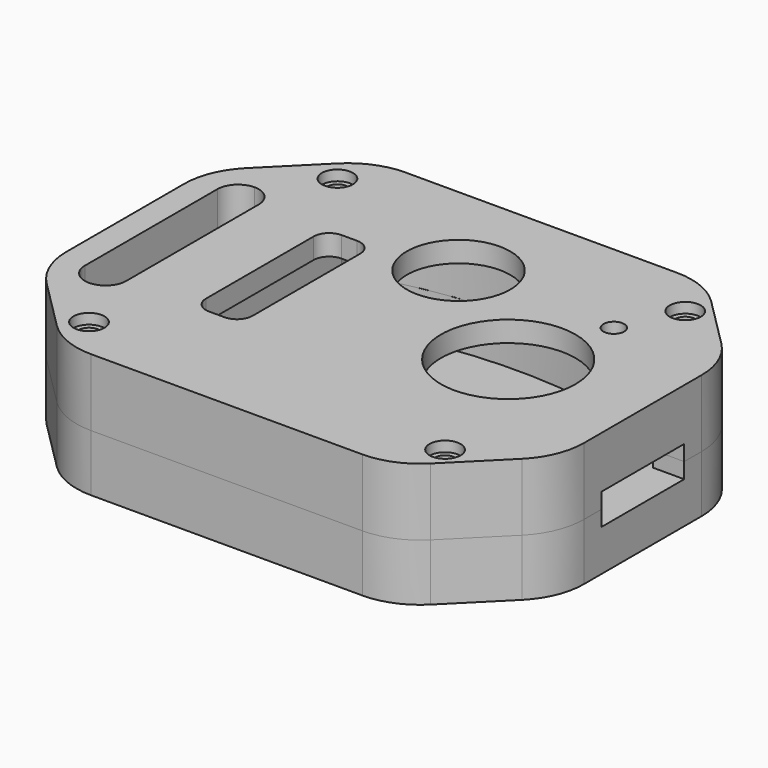
from build123d import *

# Parameters (mm, degrees)
F1_DEPTH   = 5.5
F2_DEPTH   = 1.5
F4_DEPTH   = 4.5
F5_W       = 4
F5_H       = 20
F6_DEPTH   = 25
F7_DEPTH   = 6.5
F8_DEPTH   = 1.5
F9_DEPTH   = 4.5
F10_DEPTH  = 25
F11_R      = 5
F11_R_2    = 6.5
F11_R_3    = 1
F12_DEPTH  = 4
F14_DEPTH  = 4.5
F15_SIZE   = 9
F15_2_SIZE = 9
F16_R      = 7
F16_2_R    = 7
F17_R      = 1.99999
F17_2_R    = 1.99999
F18_R      = 1
F19_DEPTH  = 7.5
F20_R      = 1.5
F20_R_2    = 1
F21_DEPTH  = 1
F22_R      = 1.5
F23_DEPTH  = 1


# Not quite as in the source:
# - a fillet or chamfer is up to 0.001 mm smaller than in the source, because OpenCascade refuses the exact size


with BuildPart() as f1:
    # F0 (on Top) → F1 (new body)
    with BuildSketch(Plane.XY):
        Polygon((25, 5), (25, 19), (-25, 19), (-25, -19), (25, -19), (25, -5), (22, -5), (22, -10), (20.5, -10), (19, -7), (19, 7), (20.5, 10), (22, 10), (22, 5), align=None)
        Polygon((25, -5), (25, 5), (22, 5), (22, 10), (20.5, 10), (19, 7), (19, -7), (20.5, -10), (22, -10), (22, -5), align=None)
    extrude(amount=-F1_DEPTH)

    # F0 (on Top) → F2 (cut)
    with BuildSketch(Plane.XY):
        Polygon((25, -5), (25, 5), (22, 5), (22, 10), (20.5, 10), (19, 7), (19, -7), (20.5, -10), (22, -10), (22, -5), align=None)
    extrude(amount=-F2_DEPTH, mode=Mode.SUBTRACT)

    # F3 (on face) → F4 (cut)
    with BuildSketch(Plane.XY):
        with BuildLine():
            Line((19, 7), (20.5, 10))
            Line((20.5, 10), (20.5, 11))
            ThreePointArc((20.5, 11), (3.1956730185, 15.4242778244), (-14.5, 13))
            Line((-14.5, 13), (-14.5, 0))
            Line((-14.5, 0), (-14.5, -13))
            ThreePointArc((-14.5, -13), (3.1956730185, -15.4242778244), (20.5, -11))
            Line((20.5, -11), (20.5, -10))
            Line((20.5, -10), (19, -7))
            Line((19, -7), (19, 7))
        make_face()
    extrude(amount=-F4_DEPTH, mode=Mode.SUBTRACT)

    # F5 (on face) → F6 (cut)
    with BuildSketch(Plane.XY):
        with Locations((-20.5, 0)):
            Rectangle(F5_W, F5_H)
    extrude(amount=-F6_DEPTH, mode=Mode.SUBTRACT)

    # F15#2
    f15_2_edges = [f1.edges().sort_by_distance(p)[0] for p in [
        (25, -19, -2.75),
        (25, 19, -2.75),
        (-25, -19, -2.75),
        (-25, 19, -2.75),
    ]]
    chamfer(f15_2_edges, length=F15_2_SIZE)

    # F16#2
    f16_2_edges = [f1.edges().sort_by_distance(p)[0] for p in [
        (16, -19, -2.75),
        (25, -10, -2.75),
        (25, 10, -2.75),
        (16, 19, -2.75),
        (-16, -19, -2.75),
        (-25, -10, -2.75),
        (-25, 10, -2.75),
        (-16, 19, -2.75),
    ]]
    fillet(f16_2_edges, radius=F16_2_R)

    # F17 (radius 2 in the source; OpenCascade refuses exactly that, so slightly less here)
    f17_edges = [f1.edges().sort_by_distance(p)[0] for p in [
        (-22.5, 10, -2.75),
        (-22.5, -10, -2.75),
        (-18.5, 10, -2.75),
        (-18.5, -10, -2.75),
    ]]
    fillet(f17_edges, radius=F17_R)


with BuildPart() as f7:
    # F0 (on Top) → F7 (new body)
    with BuildSketch(Plane.XY):
        Polygon((25, 5), (25, 19), (-25, 19), (-25, -19), (25, -19), (25, -5), (22, -5), (22, -10), (20.5, -10), (19, -7), (19, 7), (20.5, 10), (22, 10), (22, 5), align=None)
        Polygon((25, -5), (25, 5), (22, 5), (22, 10), (20.5, 10), (19, 7), (19, -7), (20.5, -10), (22, -10), (22, -5), align=None)
    extrude(amount=F7_DEPTH)

    # F0 (on Top) → F8 (cut)
    with BuildSketch(Plane.XY):
        Polygon((25, -5), (25, 5), (22, 5), (22, 10), (20.5, 10), (19, 7), (19, -7), (20.5, -10), (22, -10), (22, -5), align=None)
    extrude(amount=F8_DEPTH, mode=Mode.SUBTRACT)

    # F3 (on face) → F9 (cut)
    with BuildSketch(Plane.XY):
        with BuildLine():
            Line((19, 7), (20.5, 10))
            Line((20.5, 10), (20.5, 11))
            ThreePointArc((20.5, 11), (3.1956730185, 15.4242778244), (-14.5, 13))
            Line((-14.5, 13), (-14.5, 0))
            Line((-14.5, 0), (-14.5, -13))
            ThreePointArc((-14.5, -13), (3.1956730185, -15.4242778244), (20.5, -11))
            Line((20.5, -11), (20.5, -10))
            Line((20.5, -10), (19, -7))
            Line((19, -7), (19, 7))
        make_face()
    extrude(amount=F9_DEPTH, mode=Mode.SUBTRACT)

    # F5 (on face) → F10 (cut)
    with BuildSketch(Plane.XY):
        with Locations((-20.5, 0)):
            Rectangle(F5_W, F5_H)
    extrude(amount=F10_DEPTH, mode=Mode.SUBTRACT)

    # F11 (on face) → F12 (cut)
    with BuildSketch(Plane.XY.offset(6.5)):
        with Locations((0, 9)):
            Circle(F11_R)
        with BuildLine():
            ThreePointArc((-7.5, 6.5), (-7.9393398282, 7.5606601718), (-9, 8))
            Line((-9, 8), (-10.5, 8))
            ThreePointArc((-10.5, 8), (-11.5606601718, 7.5606601718), (-12, 6.5))
            Line((-12, 6.5), (-12, -6.5))
            ThreePointArc((-12, -6.5), (-11.5606601718, -7.5606601718), (-10.5, -8))
            Line((-10.5, -8), (-9, -8))
            ThreePointArc((-9, -8), (-7.9393398282, -7.5606601718), (-7.5, -6.5))
            Line((-7.5, -6.5), (-7.5, 6.5))
        make_face()
        with Locations((12, 0)):
            Circle(F11_R_2)
        with Locations((15, 9)):
            Circle(F11_R_3)
    extrude(amount=-F12_DEPTH, mode=Mode.SUBTRACT)

    # F13 (on face) → F14 (cut)
    with BuildSketch(Plane.XY):
        with BuildLine():
            Line((-10.6637885499, -14.1296387517), (-14.5, -13))
            ThreePointArc((-14.5, -13), (-12.5940423426, -13.6060737647), (-10.6637885499, -14.1296387517))
        make_face()
        with BuildLine():
            ThreePointArc((-10.6637885499, -14.1296387517), (-12.5940423426, -13.6060737647), (-14.5, -13))
            ThreePointArc((-14.5, -13), (-13.158992343, -15.5246230857), (-10.6637885499, -14.1296387517))
        make_face()
        with BuildLine():
            Line((19.5918852505, -11.4195493603), (15.8766396041, -12.8992627738))
            ThreePointArc((15.8766396041, -12.8992627738), (17.7501751769, -12.1993595968), (19.5918852505, -11.4195493603))
        make_face()
        with BuildLine():
            ThreePointArc((19.5918852505, -11.4195493603), (17.7501751769, -12.1993595968), (15.8766396041, -12.8992627738))
            ThreePointArc((15.8766396041, -12.8992627738), (18.4902029887, -14.0574120282), (19.5918852505, -11.4195493603))
        make_face()
        with BuildLine():
            Line((15.8766396041, 12.8992627738), (19.5918852505, 11.4195493603))
            ThreePointArc((19.5918852505, 11.4195493603), (17.7501751769, 12.1993595968), (15.8766396041, 12.8992627738))
        make_face()
        with BuildLine():
            ThreePointArc((15.8766396041, 12.8992627738), (17.7501751769, 12.1993595968), (19.5918852505, 11.4195493603))
            ThreePointArc((19.5918852505, 11.4195493603), (18.4902029887, 14.0574120282), (15.8766396041, 12.8992627738))
        make_face()
        with BuildLine():
            Line((-14.5, 13), (-10.6637885499, 14.1296387517))
            ThreePointArc((-10.6637885499, 14.1296387517), (-12.5940423426, 13.6060737647), (-14.5, 13))
        make_face()
        with BuildLine():
            ThreePointArc((-14.5, 13), (-12.5940423426, 13.6060737647), (-10.6637885499, 14.1296387517))
            ThreePointArc((-10.6637885499, 14.1296387517), (-13.158992343, 15.5246230857), (-14.5, 13))
        make_face()
    extrude(amount=F14_DEPTH, mode=Mode.SUBTRACT)

    # F15
    f15_edges = [f7.edges().sort_by_distance(p)[0] for p in [
        (25, -19, 3.25),
        (25, 19, 3.25),
        (-25, -19, 3.25),
        (-25, 19, 3.25),
    ]]
    chamfer(f15_edges, length=F15_SIZE)

    # F16
    f16_edges = [f7.edges().sort_by_distance(p)[0] for p in [
        (16, -19, 3.25),
        (25, -10, 3.25),
        (25, 10, 3.25),
        (16, 19, 3.25),
        (-16, -19, 3.25),
        (-25, -10, 3.25),
        (-25, 10, 3.25),
        (-16, 19, 3.25),
    ]]
    fillet(f16_edges, radius=F16_R)

    # F17#2 (radius 2 in the source; OpenCascade refuses exactly that, so slightly less here)
    f17_2_edges = [f7.edges().sort_by_distance(p)[0] for p in [
        (-22.5, 10, 3.25),
        (-22.5, -10, 3.25),
        (-18.5, 10, 3.25),
        (-18.5, -10, 3.25),
    ]]
    fillet(f17_2_edges, radius=F17_2_R)


with BuildPart() as f19_tool:
    # F18 (on face) → F19 (new body, symmetric)
    with BuildSketch(Plane.XY):
        with Locations((17.5, 14.5)):
            Circle(F18_R)
        with Locations((-16.5, 15)):
            Circle(F18_R)
        with Locations((-16.5, -15)):
            Circle(F18_R)
        with Locations((17.5, -14.5)):
            Circle(F18_R)
    extrude(amount=F19_DEPTH, both=True)


with BuildPart() as f1_1:
    add(f1.part)

    # F19: cut by f19_tool
    add(f19_tool.part, mode=Mode.SUBTRACT)

    # F22 (on face) → F23 (cut)
    with BuildSketch(Plane(origin=(0, 0, -5.5), x_dir=(1, 0, 0), z_dir=(0, 0, -1))):
        with Locations((-16.5, 15)):
            Circle(F22_R)
        with Locations((17.5, 14.5)):
            Circle(F22_R)
        with Locations((-16.5, -15)):
            Circle(F22_R)
        with Locations((17.5, -14.5)):
            Circle(F22_R)
    extrude(amount=-F23_DEPTH, mode=Mode.SUBTRACT)


with BuildPart() as f7_1:
    add(f7.part)

    # F19: cut by f19_tool
    add(f19_tool.part, mode=Mode.SUBTRACT)

    # F20 (on face) → F21 (cut)
    with BuildSketch(Plane.XY.offset(6.5)):
        with Locations((-16.5, -15)):
            Circle(F20_R)
        with Locations((-16.5, -15)):
            Circle(F20_R_2, mode=Mode.SUBTRACT)
        with Locations((-16.5, 15)):
            Circle(F20_R)
        with Locations((-16.5, 15)):
            Circle(F20_R_2, mode=Mode.SUBTRACT)
        with Locations((17.5, 14.5)):
            Circle(F20_R)
        with Locations((17.5, 14.5)):
            Circle(F20_R_2, mode=Mode.SUBTRACT)
        with Locations((17.5, -14.5)):
            Circle(F20_R)
        with Locations((17.5, -14.5)):
            Circle(F20_R_2, mode=Mode.SUBTRACT)
    extrude(amount=-F21_DEPTH, mode=Mode.SUBTRACT)


solid = Compound([f1_1.part, f7_1.part])
